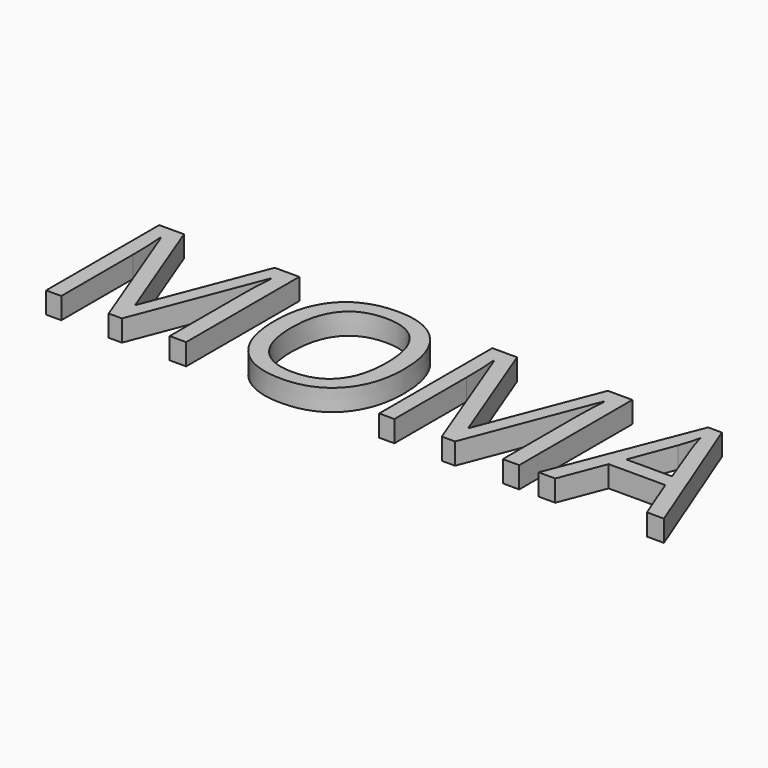
from build123d import *

# Parameters (mm, degrees)
F0_TEXT_SIZE = 27.7777777778
F1_DEPTH     = 3


# Not quite as in the source:
# - Text() gives the source's letters only with a copy of the font that has no kerning and outlines rounded to 1/6400 em; it was checked with that copy


with BuildPart() as f1:
    # F0 (on Top) → F1 (new body)
    with BuildSketch(Plane.XY):
        with Locations((0, 0)):
            Text('MOMA', F0_TEXT_SIZE, font='Open Sans', text_align=(TextAlign.LEFT, TextAlign.BOTTOM))
    extrude(amount=F1_DEPTH)


solid = f1.part
